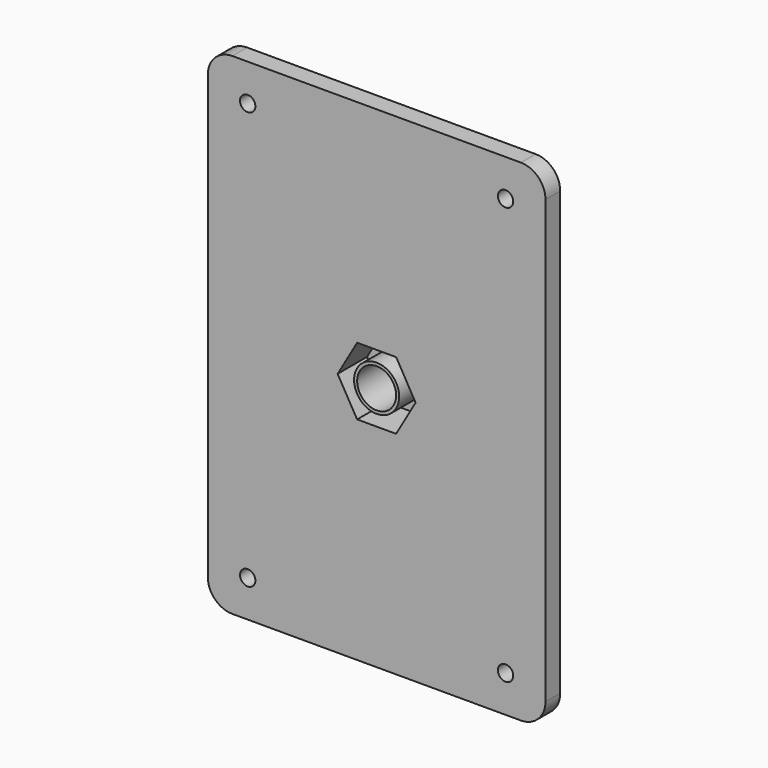
from build123d import *

# Parameters (mm, degrees)
F0_R     = 1.25
F1_DEPTH = 6
F2_R     = 1.25
F3_DEPTH = 3
F4_SIZE  = 2.99999
F5_R     = 3.175
F6_DEPTH = 3
F7_R     = 3.675
F7_R_2   = 3.175
F8_DEPTH = 6


# Not quite as in the source:
# - a fillet or chamfer is up to 0.001 mm smaller than in the source, because OpenCascade refuses the exact size


with BuildPart() as f1:
    # F0 (on Front) → F1 (new body)
    with BuildSketch(Plane.XZ):
        with BuildLine():
            Line((22.9103805721, 41.8708454072), (-24.0896194279, 41.8708454072))
            ThreePointArc((-24.0896194279, 41.8708454072), (-26.9180465527, 40.699272532), (-28.0896194279, 37.8708454072))
            Line((-28.0896194279, 37.8708454072), (-28.0896194279, -34.1291545928))
            ThreePointArc((-28.0896194279, -34.1291545928), (-26.9180465527, -36.9575817175), (-24.0896194279, -38.1291545928))
            Line((-24.0896194279, -38.1291545928), (22.9103805721, -38.1291545928))
            ThreePointArc((22.9103805721, -38.1291545928), (25.7388076968, -36.9575817175), (26.9103805721, -34.1291545928))
            Line((26.9103805721, -34.1291545928), (26.9103805721, 37.8708454072))
            ThreePointArc((26.9103805721, 37.8708454072), (25.7388076968, 40.699272532), (22.9103805721, 41.8708454072))
        make_face()
        with Locations((-21.5896194279, -32.1291545928)):
            Circle(F0_R, mode=Mode.SUBTRACT)
        with Locations((20.4103805721, -32.1291545928)):
            Circle(F0_R, mode=Mode.SUBTRACT)
        Polygon((5.7612335332, 1.8708454072), (2.5858070526, -3.6291545928), (-3.7650459085, -3.6291545928), (-6.940472389, 1.8708454072), (-3.7650459085, 7.3708454072), (2.5858070526, 7.3708454072), align=None, mode=Mode.SUBTRACT)
        with Locations((-21.5896194279, 35.8708454072)):
            Circle(F0_R, mode=Mode.SUBTRACT)
        with Locations((20.4103805721, 35.8708454072)):
            Circle(F0_R, mode=Mode.SUBTRACT)
    extrude(amount=F1_DEPTH)

    # F2 (on face) → F3 (cut)
    with BuildSketch(Plane(origin=(0, 0, 0), x_dir=(-1, 0, 0), z_dir=(0, 1, 0))):
        with BuildLine():
            ThreePointArc((28.0896194279, 37.8708454072), (26.9180465527, 40.699272532), (24.0896194279, 41.8708454072))
            Line((24.0896194279, 41.8708454072), (-22.9103805721, 41.8708454072))
            ThreePointArc((-22.9103805721, 41.8708454072), (-25.7388076968, 40.699272532), (-26.9103805721, 37.8708454072))
            Line((-26.9103805721, 37.8708454072), (-26.9103805721, -34.1291545928))
            ThreePointArc((-26.9103805721, -34.1291545928), (-25.7388076968, -36.9575817175), (-22.9103805721, -38.1291545928))
            Line((-22.9103805721, -38.1291545928), (24.0896194279, -38.1291545928))
            ThreePointArc((24.0896194279, -38.1291545928), (26.9180465527, -36.9575817175), (28.0896194279, -34.1291545928))
            Line((28.0896194279, -34.1291545928), (28.0896194279, 37.8708454072))
        make_face()
        with Locations((-20.4103805721, -32.1291545928)):
            Circle(F2_R, mode=Mode.SUBTRACT)
        with Locations((21.5896194279, -32.1291545928)):
            Circle(F2_R, mode=Mode.SUBTRACT)
        Polygon((13.2913253501, 1.8708454072), (6.940472389, -9.1291545928), (-5.7612335332, -9.1291545928), (-12.1120864943, 1.8708454072), (-5.7612335332, 12.8708454072), (6.940472389, 12.8708454072), align=None, mode=Mode.SUBTRACT)
        with Locations((-20.4103805721, 35.8708454072)):
            Circle(F2_R, mode=Mode.SUBTRACT)
        with Locations((21.5896194279, 35.8708454072)):
            Circle(F2_R, mode=Mode.SUBTRACT)
    extrude(amount=-F3_DEPTH, mode=Mode.SUBTRACT)

    # F4 (size 3 in the source; OpenCascade refuses exactly that, so slightly less here)
    f4_edges = [f1.edges().sort_by_distance(p)[0] for p in [
        (8.93666, -3, 7.370845),
        (8.93666, -3, -3.629155),
        (-0.589619, -3, -9.129155),
        (-10.115899, -3, -3.629155),
        (-10.115899, -3, 7.370845),
        (-0.589619, -3, 12.870845),
    ]]
    chamfer(f4_edges, length=F4_SIZE)

    # F5 (on face) → F6 (join)
    with BuildSketch(Plane(origin=(0, 0, 0), x_dir=(-1, 0, 0), z_dir=(0, 1, 0))):
        Polygon((6.940472389, -9.1291545928), (13.2913253501, 1.8708454072), (6.940472389, 12.8708454072), (-5.7612335332, 12.8708454072), (-12.1120864943, 1.8708454072), (-5.7612335332, -9.1291545928), align=None)
        Polygon((3.7650459085, -3.6291545928), (-2.5858070526, -3.6291545928), (-5.7612335332, 1.8708454072), (-2.5858070526, 7.3708454072), (3.7650459085, 7.3708454072), (6.940472389, 1.8708454072), align=None, mode=Mode.SUBTRACT)
        Polygon((-5.7612335332, 1.8708454072), (-2.5858070526, -3.6291545928), (3.7650459085, -3.6291545928), (6.940472389, 1.8708454072), (3.7650459085, 7.3708454072), (-2.5858070526, 7.3708454072), align=None)
        with Locations((0.5896194279, 1.8708454072)):
            Circle(F5_R, mode=Mode.SUBTRACT)
    extrude(amount=F6_DEPTH)

    # F7 (on face) → F8 (join, through all)
    with BuildSketch(Plane.XZ):
        with Locations((-0.5896194279, 1.8708454072)):
            Circle(F7_R)
        with Locations((-0.5896194279, 1.8708454072)):
            Circle(F7_R_2, mode=Mode.SUBTRACT)
    extrude(amount=F8_DEPTH)


solid = f1.part
